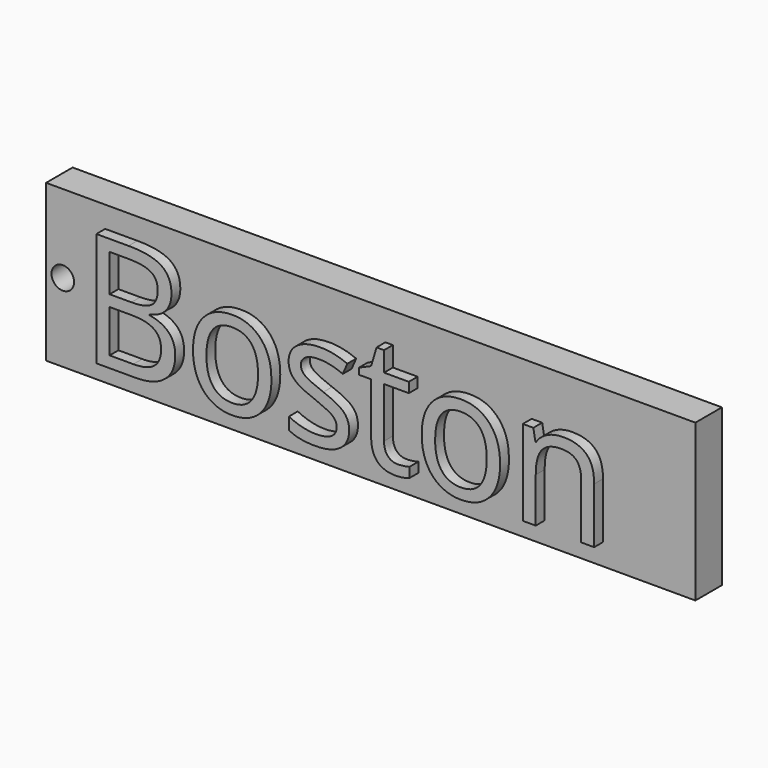
from build123d import *

# Parameters (mm, degrees)
F0_W         = 89.5075909793
F0_H         = 21.5854314156
F1_DEPTH     = 4.572
F2_R         = 1.5565479364
F3_DEPTH     = 70.104
F4_TEXT_SIZE = 21.9851615839
F5_DEPTH     = 1.524


# Not quite as in the source:
# - Text() gives the source's letters only with a copy of the font that has no kerning and outlines rounded to 1/6400 em; it was checked with that copy


with BuildPart() as f1:
    # F0 (on Front) → F1 (new body)
    with BuildSketch(Plane.XZ):
        with Locations((-6.9073382765, -3.1658632215)):
            Rectangle(F0_W, F0_H)
    extrude(amount=F1_DEPTH)

    # F2 (on face) → F3 (cut)
    with BuildSketch(Plane.XZ.offset(4.572)):
        with Locations((-49.3586882949, -3.1658632215)):
            Circle(F2_R)
    extrude(amount=-F3_DEPTH, mode=Mode.SUBTRACT)

    # F4 (on face) → F5 (join)
    with BuildSketch(Plane.XZ.offset(4.572)):
        with Locations((-45.6677377224, -11.0105350614)):
            Text('Boston', F4_TEXT_SIZE, font='Open Sans', text_align=(TextAlign.LEFT, TextAlign.BOTTOM))
    extrude(amount=F5_DEPTH)


solid = f1.part
